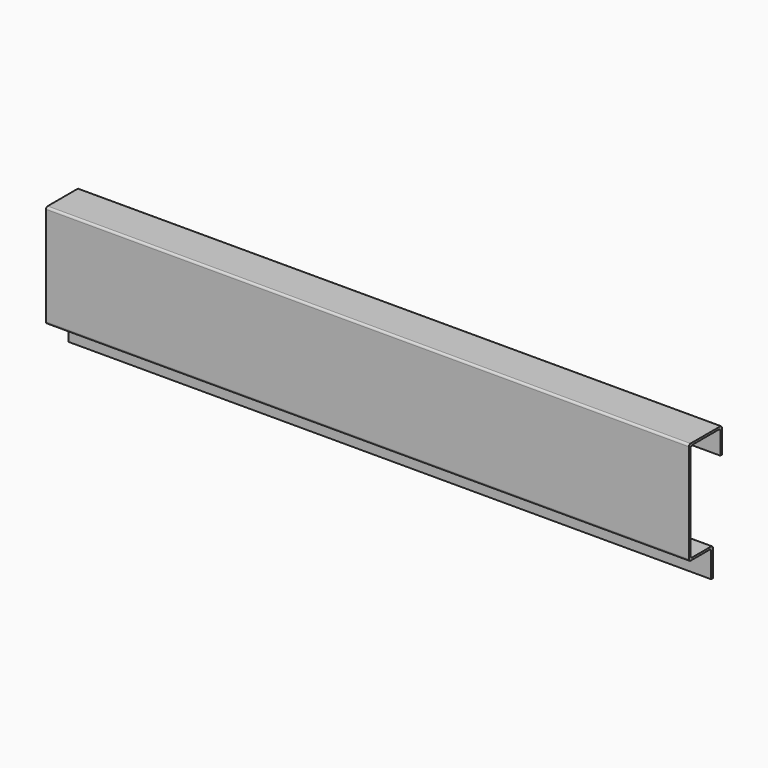
from build123d import *

# Parameters (mm, degrees)
F1_DEPTH = 623
F3_D     = 5
F4_R     = 2


# Not quite as in the source:
# - a feature names something its author has since deleted; it is built from what else it names


with BuildPart() as f1:
    # F0 (on Right) → F1 (new body)
    with BuildSketch(Plane.YZ):
        Polygon((-18.8378913403, 177.8021101952), (-18.8378913403, 154.8021101952), (-16.8378913403, 154.8021101952), (-16.8378913403, 179.8021101952), (-56.8378913403, 179.8021101952), (-56.8378913403, 79.8021101952), (-29.8378913403, 79.8021101952), (-29.8378913403, 53.8021101952), (-27.8378913403, 53.8021101952), (-27.8378913403, 81.8021101952), (-54.8378913403, 81.8021101952), (-54.8378913403, 177.8021101952), align=None)
    extrude(amount=F1_DEPTH)

    # F3 (through all)
    with Locations(Plane.XZ.offset(29.8378913403)):
        with Locations((523, 66.8021101952), (100, 66.8021101952)):
            Hole(F3_D / 2)

    # F4
    f4_edges = [f1.edges().sort_by_distance(p)[0] for p in [
        (311.5, -56.837891, 179.80211),
        (311.5, -16.837891, 179.80211),
        (311.5, -56.837891, 79.80211),
        (311.5, -27.837891, 81.80211),
        (311.5, -54.837891, 81.80211),
        (311.5, -29.837891, 79.80211),
        (311.5, -18.837891, 177.80211),
        (311.5, -54.837891, 177.80211),
    ]]
    fillet(f4_edges, radius=F4_R)


solid = f1.part
